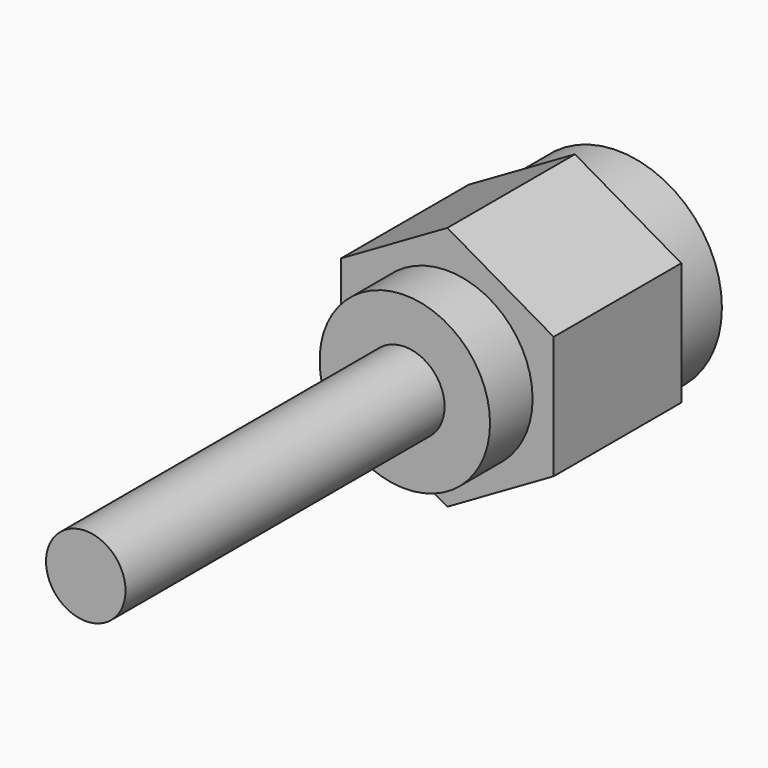
from build123d import *

# Parameters (mm, degrees)
F0_R     = 1.495231247
F1_DEPTH = 25
F2_START = 2
F0_R_2   = 3.9260289208
F2_DEPTH = 6
F3_START = 4
F0_R_3   = 3.2049719045
F3_DEPTH = 6
F4_DEPTH = 8


with BuildPart() as f1:
    # F0 (on Front) → F1 (new body)
    with BuildSketch(Plane.XZ):
        Circle(F0_R)
    extrude(amount=F1_DEPTH)

    # F0 (on Front) → F3 (join)
    with BuildSketch(Plane.XZ.offset(F3_START)):
        Circle(F0_R_3)
        Circle(F0_R, mode=Mode.SUBTRACT)
    extrude(amount=F3_DEPTH)


with BuildPart() as f2:
    # F0 (on Front) → F2 (new body)
    with BuildSketch(Plane.XZ.offset(F2_START)):
        Polygon((3.997805994, -2.3081343668), (3.997805994, 2.3081343668), (0, 4.6162687336), (-3.997805994, 2.3081343668), (-3.997805994, -2.3081343668), (0, -4.6162687336), align=None)
        Circle(F0_R_2, mode=Mode.SUBTRACT)
    extrude(amount=F2_DEPTH)

    # F0 (on Front) → F4 (join)
    with BuildSketch(Plane.XZ):
        Circle(F0_R_2)
        Circle(F0_R_3, mode=Mode.SUBTRACT)
    extrude(amount=F4_DEPTH)


solid = Compound([f1.part, f2.part])
